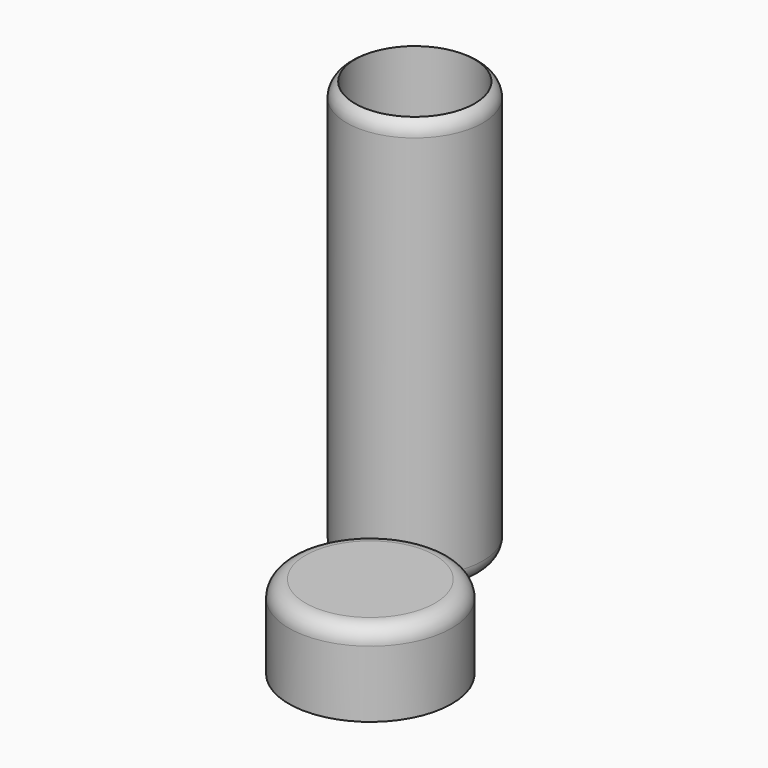
from build123d import *

# Parameters (mm, degrees)
F0_R     = 20.8011529173
F1_DEPTH = 127
F2_T     = -2.54
F4_R     = 24.8400420573
F5_DEPTH = 25.4
F6_R     = 5.08
F7_T     = -2.54


# Not quite as in the source:
# - a fillet or chamfer that OpenCascade refuses, or shapes differently, is made with other operations: its cross-section is extruded or revolved along the edge and cut away or added


with BuildPart() as f1:
    # F0 (on Top) → F1 (new body)
    with BuildSketch(Plane.XY):
        Circle(F0_R)
    extrude(amount=F1_DEPTH)

    # F2
    f2_openings = [f1.faces().sort_by_distance(p)[0] for p in [
        (0, 0, 127),
    ]]
    offset(amount=F2_T, openings=f2_openings)

    # F3: fillet of radius 5.08 on 3 edges, made by hand

    # F3_s1 → F3_t2 (revolve, cut)
    with BuildSketch(Plane.XZ):
        with BuildLine():
            ThreePointArc((20.8013029173, 5.07985), (19.3134053657, 1.4877475516), (15.7213029173, -0.00015))
            Line((15.7213029173, -0.00015), (15.7213029173, -0.10175))
            ThreePointArc((15.7213029173, -0.10175), (18.2612279173, -0.1016), (20.8011529173, -0.1016))
            Line((20.8011529173, -0.1016), (20.9027529173, 0))
            ThreePointArc((20.9027529173, 0), (20.9027529173, 2.539925), (20.9029029173, 5.07985))
            Line((20.9029029173, 5.07985), (20.8013029173, 5.07985))
        make_face()
    revolve(axis=Axis((0, 0, 0), (0, 0, 1)), mode=Mode.SUBTRACT)

    # F3_s3 → F3_t4 (revolve, cut)
    with BuildSketch(Plane.XZ):
        with BuildLine():
            ThreePointArc((20.8013029173, 122.6006775522), (20.1206903172, 125.140715053), (18.2612279151, 127.0001299051))
            Line((18.2612279151, 127.0001299051), (18.312026415, 127.0881189521))
            ThreePointArc((18.312026415, 127.0881189521), (19.5311904162, 127.1016), (20.8011529173, 127.1016))
            Line((20.8011529173, 127.1016), (20.9027529173, 127))
            ThreePointArc((20.9027529173, 127), (20.9027529173, 124.8003387761), (20.9029029173, 122.6006775522))
            Line((20.9029029173, 122.6006775522), (20.8013029173, 122.6006775522))
        make_face()
    revolve(axis=Axis((0, 0, 127), (0, 0, 1)), mode=Mode.SUBTRACT)


with BuildPart() as f5:
    # F4 (on Top) → F5 (new body)
    with BuildSketch(Plane.XY):
        with Locations((30.1989763975, -54.7148250043)):
            Circle(F4_R)
    extrude(amount=F5_DEPTH)

    # F6
    f6_edges = [f5.edges().sort_by_distance(p)[0] for p in [
        (5.358934, -54.714825, 25.4),
    ]]
    fillet(f6_edges, radius=F6_R)

    # F7
    f7_openings = [f5.faces().sort_by_distance(p)[0] for p in [
        (30.198976, -54.714825, 0),
    ]]
    offset(amount=F7_T, openings=f7_openings)


solid = Compound([f1.part, f5.part])
